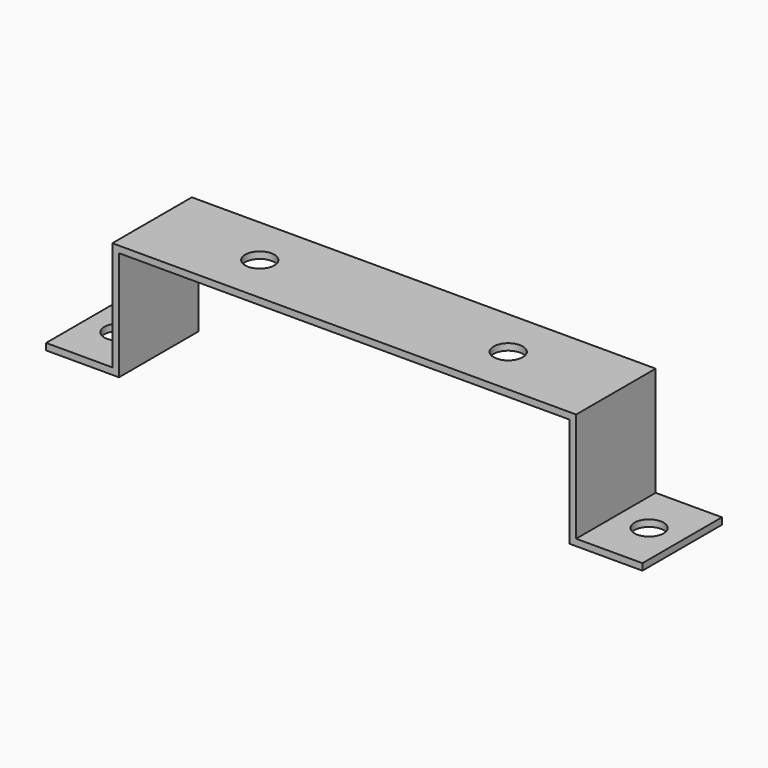
from build123d import *

# Parameters (mm, degrees)
F1_DEPTH = 30
F2_R     = 4.4
F3_R     = 4.4
F4_DEPTH = 25


# Not quite as in the source:
# - a feature names something its author has since deleted; it is built from what else it names


with BuildPart() as f1:
    # F0 (on Front) → F1 (new body)
    with BuildSketch(Plane.XZ):
        Polygon((90, -1), (90, 1), (70, 1), (70, 34), (-70, 34), (-70, 1), (-90, 1), (-90, -1), (-68, -1), (-68, 32), (68, 32), (68, -1), align=None)
    extrude(amount=F1_DEPTH)

    # F2 (on face) + F3 (on face) → F4 (cut)
    with BuildSketch(Plane.XY.offset(1)):
        with Locations((-80, -15)):
            Circle(F2_R)
        with Locations((80, -15)):
            Circle(F2_R)
    with BuildSketch(Plane.XY.offset(34)):
        with Locations((-37.5, -15)):
            Circle(F3_R)
        with Locations((37.5, -15)):
            Circle(F3_R)
    extrude(amount=-F4_DEPTH, mode=Mode.SUBTRACT)


solid = f1.part
